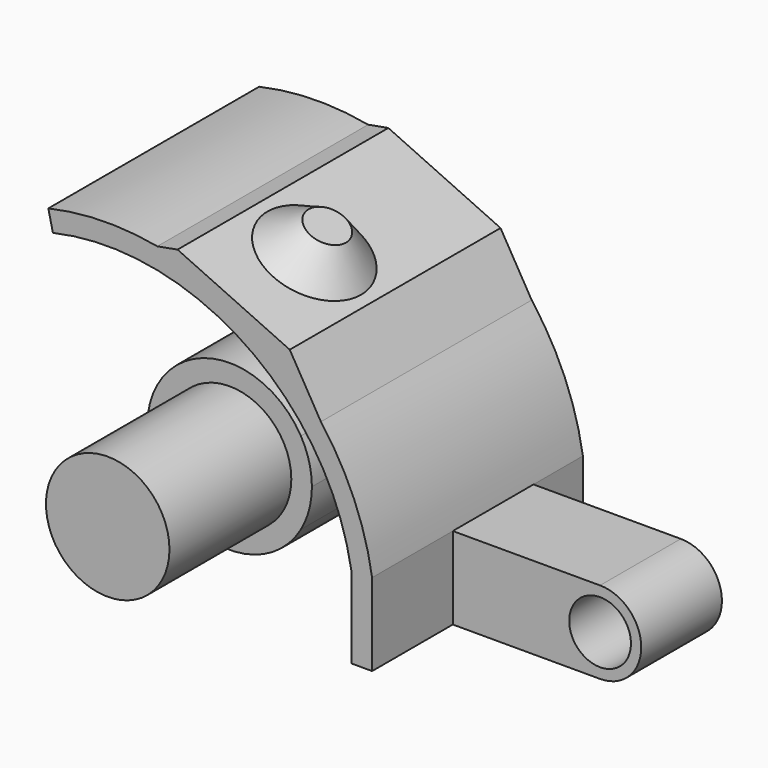
from build123d import *

# Parameters (mm, degrees)
F0_W      = 1.0130730125
F0_H      = 4
F1_DEPTH  = 9.8
F0_R      = 3
F2_DEPTH  = 3
F0_W_2    = 2
F0_R_2    = 1.5
F3_DEPTH  = 4.9
F4_R      = 3
F5_DEPTH  = 9.8
F6_DEPTH  = 2.4
F7_R      = 2.5
F8_DEPTH  = 1.5
F9_SIZE   = 1.49999
F10_DEPTH = 3


# Not quite as in the source:
# - a fillet or chamfer is up to 0.001 mm smaller than in the source, because OpenCascade refuses the exact size
# - a feature names something its author has since deleted; it is built from what else it names


with BuildPart() as f1:
    # F0 (on Front) → F1 (new body)
    with BuildSketch(Plane.XZ):
        with BuildLine():
            ThreePointArc((-2.6630696544, 11.7007717701), (6.6741513084, 9.9727480823), (11.8321595662, 2))
            Line((11.8321595662, 2), (12.8452325787, 2))
            ThreePointArc((12.8452325787, 2), (11.9653059951, 5.0824651934), (10.3578419044, 7.8558965804))
            ThreePointArc((10.3578419044, 7.8558965804), (6.8410523386, 11.0544110156), (2.4094924969, 12.7747542406))
            ThreePointArc((2.4094924969, 12.7747542406), (-0.2428398127, 12.99773168), (-2.8849921256, 12.6758360843))
            Line((-2.8849921256, 12.6758360843), (-2.6630696544, 11.7007717701))
        make_face()
        with Locations((12.3386960724, 0)):
            Rectangle(F0_W, F0_H)
        with BuildLine():
            ThreePointArc((2.4094924969, 12.7747542406), (6.8410523386, 11.0544110156), (10.3578419044, 7.8558965804))
            Line((10.3578419044, 7.8558965804), (8.8443472742, 10.4461347942))
            Line((8.8443472742, 10.4461347942), (3.3933836255, 12.9535229374))
            Line((3.3933836255, 12.9535229374), (2.4094924969, 12.7747542406))
        make_face()
    extrude(amount=F1_DEPTH)

    # F0 (on Front) → F2 (join)
    with BuildSketch(Plane.XZ):
        with Locations((12.3386960724, 0)):
            Rectangle(F0_W, F0_H)
        with BuildLine():
            Line((11.8321595662, 2), (3.4641016151, 2))
            ThreePointArc((3.4641016151, 2), (3.8637033052, 1.0352761804), (4, 0))
            ThreePointArc((4, 0), (3.8637033052, -1.0352761804), (3.4641016151, -2))
            Line((3.4641016151, -2), (11.8321595662, -2))
            Line((11.8321595662, -2), (11.8321595662, 2))
        make_face()
        with BuildLine():
            ThreePointArc((4, 0), (3.8637033052, 1.0352761804), (3.4641016151, 2))
            ThreePointArc((3.4641016151, 2), (-4, 0), (3.4641016151, -2))
            ThreePointArc((3.4641016151, -2), (3.8637033052, -1.0352761804), (4, 0))
        make_face()
        Circle(F0_R, mode=Mode.SUBTRACT)
        Circle(F0_R)
    extrude(amount=-F2_DEPTH)

    # F0 (on Front) → F3 (join)
    with BuildSketch(Plane.XZ):
        with Locations((13.8452325787, 0)):
            Rectangle(F0_W_2, F0_H)
        with BuildLine():
            Line((20, 2), (14.8452325787, 2))
            Line((14.8452325787, 2), (14.8452325787, -2))
            Line((14.8452325787, -2), (20, -2))
            ThreePointArc((20, -2), (22, 0), (20, 2))
        make_face()
        with Locations((20, 0)):
            Circle(F0_R_2, mode=Mode.SUBTRACT)
    extrude(amount=F3_DEPTH)

    # F4 (on face) → F5 (join)
    with BuildSketch(Plane.XZ):
        Circle(F4_R)
    extrude(amount=F5_DEPTH)

    # F4 (on face) → F6 (join)
    with BuildSketch(Plane.XZ):
        with BuildLine():
            ThreePointArc((3.4641016151, -2), (3.8637033052, -1.0352761804), (4, 0))
            ThreePointArc((4, 0), (3.8637033052, 1.0352761804), (3.4641016151, 2))
            ThreePointArc((3.4641016151, 2), (-4, 0), (3.4641016151, -2))
        make_face()
        Circle(F4_R, mode=Mode.SUBTRACT)
    extrude(amount=F6_DEPTH)

    # F7 (on face) → F8 (join)
    with BuildSketch(Plane(origin=(5.5105226193, 0, 11.9796604147), x_dir=(0.9084939414, 0, -0.4178980239), z_dir=(0.4178980239, 0, 0.9084939414))):
        with Locations((0.6696168272, -4.9)):
            Circle(F7_R)
    extrude(amount=F8_DEPTH)

    # F9 (size 1.5 in the source; OpenCascade refuses exactly that, so slightly less here)
    f9_edges = [f1.edges().sort_by_distance(p)[0] for p in [
        (4.474478, -4.9, 14.107315),
    ]]
    chamfer(f9_edges, length=F9_SIZE)

    # F10 (add): a face of the model
    f10_faces = [f1.faces().sort_by_distance(p)[0] for p in [
        (-0.2392542287, 0, 12.8058172707),
    ]]
    extrude(f10_faces, amount=F10_DEPTH)


solid = f1.part
